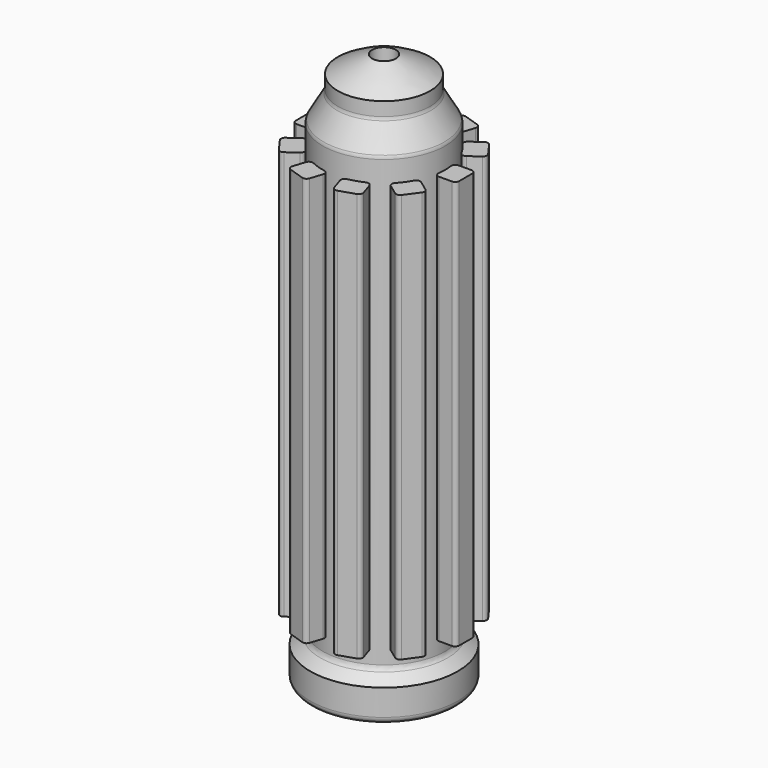
from build123d import *

# Parameters (mm, degrees)
F2_R     = 1.6
F4_W     = 6
F4_H     = 100
F6_R     = 1
F7_COUNT = 10


with BuildPart() as f1:
    # F0 (on Front) → F1 (revolve)
    with BuildSketch(Plane.XZ):
        with BuildLine():
            ThreePointArc((11.2808425035, 130.7535704158), (7.1652289239, 133.0216140638), (2.902801656, 135))
            Line((2.902801656, 135), (2.902801656, 125))
            Line((2.902801656, 125), (10.75, 125))
            Line((10.75, 125), (10.75, 0))
            Line((10.75, 0), (18.0487800966, 0))
            Line((18.0487800966, 0), (18.0487800966, 8))
            Line((18.0487800966, 8), (15, 10.5582302546))
            Line((15, 10.5582302546), (15, 120.5582302546))
            Line((15, 120.5582302546), (11.2808425035, 127))
            Line((11.2808425035, 127), (11.2808425035, 130.7535704158))
        make_face()
    revolve(axis=Axis((0, 0, 37.109490484), (0, 0, 1)))

    # F2
    f2_edges = [f1.edges().sort_by_distance(p)[0] for p in [
        (-15, 0, 120.55823),
        (-11.280843, 0, 127),
        (-18.04878, 0, 0),
        (-15, 0, 10.55823),
    ]]
    fillet(f2_edges, radius=F2_R)


with BuildPart() as f5:
    # F4 (on offset) → F5 (new body, up to the next surface of F1)
    with BuildSketch(Plane.YZ.offset(20)):
        with Locations((0, 65)):
            Rectangle(F4_W, F4_H)
    extrude(until=Until.NEXT, target=f1.part, dir=(-1, 0, 0))

    # F6
    f6_edges = [f5.edges().sort_by_distance(p)[0] for p in [
        (20, -3, 65),
        (20, 3, 65),
        (14.696938, 3, 65),
        (14.696938, -3, 65),
    ]]
    fillet(f6_edges, radius=F6_R)


with BuildPart() as f7_1:
    # F7: instance of F5
    add(f5.part.rotate(Axis((0, 0, 10.5582302546), (0, 0, -1)), 1 * 360 / F7_COUNT))


with BuildPart() as f7_2:
    # F7: instance of F5
    add(f5.part.rotate(Axis((0, 0, 10.5582302546), (0, 0, -1)), 2 * 360 / F7_COUNT))


with BuildPart() as f7_3:
    # F7: instance of F5
    add(f5.part.rotate(Axis((0, 0, 10.5582302546), (0, 0, -1)), 3 * 360 / F7_COUNT))


with BuildPart() as f7_4:
    # F7: instance of F5
    add(f5.part.rotate(Axis((0, 0, 10.5582302546), (0, 0, -1)), 4 * 360 / F7_COUNT))


with BuildPart() as f7_5:
    # F7: instance of F5
    add(f5.part.rotate(Axis((0, 0, 10.5582302546), (0, 0, -1)), 5 * 360 / F7_COUNT))


with BuildPart() as f7_6:
    # F7: instance of F5
    add(f5.part.rotate(Axis((0, 0, 10.5582302546), (0, 0, -1)), 6 * 360 / F7_COUNT))


with BuildPart() as f7_7:
    # F7: instance of F5
    add(f5.part.rotate(Axis((0, 0, 10.5582302546), (0, 0, -1)), 7 * 360 / F7_COUNT))


with BuildPart() as f7_8:
    # F7: instance of F5
    add(f5.part.rotate(Axis((0, 0, 10.5582302546), (0, 0, -1)), 8 * 360 / F7_COUNT))


with BuildPart() as f7_9:
    # F7: instance of F5
    add(f5.part.rotate(Axis((0, 0, 10.5582302546), (0, 0, -1)), 9 * 360 / F7_COUNT))


solid = Compound([f1.part, f5.part, f7_1.part, f7_2.part, f7_3.part, f7_4.part, f7_5.part, f7_6.part, f7_7.part, f7_8.part, f7_9.part])
